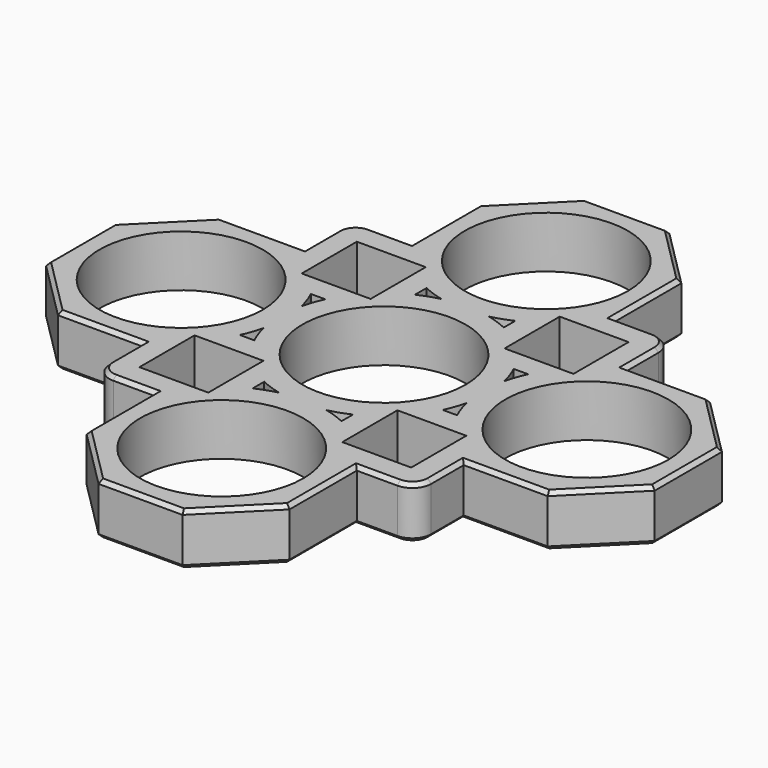
from build123d import *

# Parameters (mm, degrees)
F0_R         = 11.0109
F1_DEPTH     = 6.985
F2_W         = 9.299216499
F2_H         = 9.299216499
F3_DEPTH     = 25.4
F4_R         = 2.54
F5_SIZE      = 0.508
F6_SIZE      = 0.508
F7_T         = 3.048
F7_T3_DEPTH  = 12.065
F7_T5_DEPTH  = 6.9758818102
F7_T7_DEPTH  = 6.9758818102
F7_T9_DEPTH  = 6.9758818102
F7_T11_DEPTH = 6.9758818102
F7_T13_DEPTH = 6.9758818102
F7_T15_DEPTH = 13.081
F7_T17_DEPTH = 6.9758818102
F7_T19_DEPTH = 6.9758818102
F7_T21_DEPTH = 6.9758818102


# Not quite as in the source:
# - a shell that OpenCascade refuses in one call is made with other operations: the cavity is built on its own and cut out


with BuildPart() as f1:
    # F0 (on Top) → F1 (new body)
    with BuildSketch(Plane.XY):
        Polygon((-13.6927261634, 5.6717128827), (-13.6927261634, -5.6717128827), (-21.7137394441, -13.6927261634), (-21.7137394441, -21.7137394441), (-13.6927261634, -21.7137394441), (-5.6717128827, -13.6927261634), (5.6717128827, -13.6927261634), (13.6927261634, -21.7137394441), (21.7137394441, -21.7137394441), (21.7137394441, -13.6927261634), (13.6927261634, -5.6717128827), (13.6927261634, 5.6717128827), (21.7137394441, 13.6927261634), (21.7137394441, 21.7137394441), (13.6927261634, 21.7137394441), (5.6717128827, 13.6927261634), (-5.6717128827, 13.6927261634), (-13.6927261634, 21.7137394441), (-21.7137394441, 21.7137394441), (-21.7137394441, 13.6927261634), align=None)
        Circle(F0_R, mode=Mode.SUBTRACT)
        Polygon((-21.7137394441, -13.6927261634), (-13.6927261634, -5.6717128827), (-13.6927261634, 5.6717128827), (-21.7137394441, 13.6927261634), (-33.0571652095, 13.6927261634), (-41.0781784902, 5.6717128827), (-41.0781784902, -5.6717128827), (-33.0571652095, -13.6927261634), align=None)
        with Locations((-27.3854523268, 0)):
            Circle(F0_R, mode=Mode.SUBTRACT)
        Polygon((-5.6717128827, -13.6927261634), (-13.6927261634, -21.7137394441), (-13.6927261634, -33.0571652095), (-5.6717128827, -41.0781784902), (5.6717128827, -41.0781784902), (13.6927261634, -33.0571652095), (13.6927261634, -21.7137394441), (5.6717128827, -13.6927261634), align=None)
        with Locations((0, -27.3854523268)):
            Circle(F0_R, mode=Mode.SUBTRACT)
        Polygon((-13.6927261634, 33.0571652095), (-13.6927261634, 21.7137394441), (-5.6717128827, 13.6927261634), (5.6717128827, 13.6927261634), (13.6927261634, 21.7137394441), (13.6927261634, 33.0571652095), (5.6717128827, 41.0781784902), (-5.6717128827, 41.0781784902), align=None)
        with Locations((0, 27.3854523268)):
            Circle(F0_R, mode=Mode.SUBTRACT)
        Polygon((13.6927261634, -5.6717128827), (21.7137394441, -13.6927261634), (33.0571652095, -13.6927261634), (41.0781784902, -5.6717128827), (41.0781784902, 5.6717128827), (33.0571652095, 13.6927261634), (21.7137394441, 13.6927261634), (13.6927261634, 5.6717128827), align=None)
        with Locations((27.3854523268, 0)):
            Circle(F0_R, mode=Mode.SUBTRACT)
    extrude(amount=-F1_DEPTH)

    # F2 (on Top) → F3 (cut)
    with BuildSketch(Plane.XY):
        with Locations((-13.6927261634, 13.6927261634)):
            Rectangle(F2_W, F2_H)
        with Locations((13.6927261634, 13.6927261634)):
            Rectangle(F2_W, F2_H)
        with Locations((13.6927261634, -13.6927261634)):
            Rectangle(F2_W, F2_H)
        with Locations((-13.6927261634, -13.6927261634)):
            Rectangle(F2_W, F2_H)
    extrude(amount=-F3_DEPTH, mode=Mode.SUBTRACT)

    # F4
    f4_edges = [f1.edges().sort_by_distance(p)[0] for p in [
        (-21.713739, 21.713739, -3.4925),
        (21.713739, 21.713739, -3.4925),
        (21.713739, -21.713739, -3.4925),
        (-21.713739, -21.713739, -3.4925),
    ]]
    fillet(f4_edges, radius=F4_R)

    # F5
    f5_edges = [f1.edges().sort_by_distance(p)[0] for p in [
        (41.078178, 0, -6.985),
        (37.067672, 9.68222, -6.985),
        (27.385452, 13.692726, -6.985),
        (21.713739, 16.433233, -6.985),
        (16.433233, 21.713739, -6.985),
        (13.692726, 27.385452, -6.985),
        (9.68222, 37.067672, -6.985),
        (0, 41.078178, -6.985),
        (-9.68222, 37.067672, -6.985),
        (-13.692726, 27.385452, -6.985),
        (-16.433233, 21.713739, -6.985),
        (37.067672, -9.68222, -6.985),
        (27.385452, -13.692726, -6.985),
        (21.713739, -16.433233, -6.985),
        (16.433233, -21.713739, -6.985),
        (13.692726, -27.385452, -6.985),
        (9.68222, -37.067672, -6.985),
        (0, -41.078178, -6.985),
        (-9.68222, -37.067672, -6.985),
        (-13.692726, -27.385452, -6.985),
        (-16.433233, -21.713739, -6.985),
        (-21.713739, -16.433233, -6.985),
        (-27.385452, -13.692726, -6.985),
        (-37.067672, -9.68222, -6.985),
        (-41.078178, 0, -6.985),
        (-37.067672, 9.68222, -6.985),
        (-27.385452, 13.692726, -6.985),
        (-21.713739, 16.433233, -6.985),
    ]]
    chamfer(f5_edges, length=F5_SIZE)

    # F6
    f6_edges = [f1.edges().sort_by_distance(p)[0] for p in [
        (9.68222, -37.067672, 0),
        (0, -41.078178, 0),
        (-9.68222, -37.067672, 0),
        (-13.692726, -27.385452, 0),
        (-16.433233, -21.713739, 0),
        (-21.713739, -16.433233, 0),
        (-27.385452, -13.692726, 0),
        (-37.067672, -9.68222, 0),
        (-27.385452, 13.692726, 0),
        (-37.067672, 9.68222, 0),
        (-41.078178, 0, 0),
        (-21.713739, 16.433233, 0),
        (-16.433233, 21.713739, 0),
        (-13.692726, 27.385452, 0),
        (-9.68222, 37.067672, 0),
        (0, 41.078178, 0),
        (9.68222, 37.067672, 0),
        (13.692726, 27.385452, 0),
        (16.433233, 21.713739, 0),
        (21.713739, 16.433233, 0),
        (27.385452, 13.692726, 0),
        (37.067672, 9.68222, 0),
        (41.078178, 0, 0),
        (37.067672, -9.68222, 0),
        (27.385452, -13.692726, 0),
        (21.713739, -16.433233, 0),
        (16.433233, -21.713739, 0),
        (13.692726, -27.385452, 0),
    ]]
    chamfer(f6_edges, length=F6_SIZE)

    # F7: shell of thickness 3.048, made by hand


with BuildPart() as f7_core1:
    # F7_t2: copy of F1
    add(f1.part)

    # the walls: a layer under each face that stays
    f7_faces = [f7_core1.faces().sort_by_distance(p)[0] for p in [
        (21.7137394441, 16.4332328037, -3.4925),
        (21.4597394441, 16.1792328037, -0.254),
        (21.4597394441, 16.1792328037, -6.731),
        (27.3854523268, 13.6927261634, -3.4925),
        (20.7901855458, 20.7901855458, -0.254),
        (20.7901855458, 20.7901855458, -6.731),
        (16.4332328037, 21.7137394441, -3.4925),
        (27.1314523268, 13.4387261634, -0.254),
        (27.1314523268, 13.4387261634, -6.731),
        (37.0676718499, 9.6822195231, -3.4925),
        (16.1792328037, 21.4597394441, -0.254),
        (16.1792328037, 21.4597394441, -6.731),
        (13.6927261634, 27.3854523268, -3.4925),
        (36.8880667274, 9.5026144006, -0.254),
        (9.5026144006, -36.8880667274, -0.254),
        (0, -40.8241784902, -0.254),
        (13.4387261634, -27.1314523268, -0.254),
        (-9.5026144006, -36.8880667274, -0.254),
        (16.1792328037, -21.4597394441, -0.254),
        (-13.4387261634, -27.1314523268, -0.254),
        (20.7901855458, -20.7901855458, -0.254),
        (-16.1792328037, -21.4597394441, -0.254),
        (21.4597394441, -16.1792328037, -0.254),
        (-20.7901855458, -20.7901855458, -0.254),
        (27.1314523268, -13.4387261634, -0.254),
        (-21.4597394441, -16.1792328037, -0.254),
        (36.8880667274, -9.5026144006, -0.254),
        (-27.1314523268, -13.4387261634, -0.254),
        (40.8241784902, 0, -0.254),
        (-36.8880667274, -9.5026144006, -0.254),
        (-40.8241784902, 0, -0.254),
        (-36.8880667274, 9.5026144006, -0.254),
        (-27.1314523268, 13.4387261634, -0.254),
        (-21.4597394441, 16.1792328037, -0.254),
        (-20.7901855458, 20.7901855458, -0.254),
        (13.4387261634, 27.1314523268, -0.254),
        (-16.1792328037, 21.4597394441, -0.254),
        (9.5026144006, 36.8880667274, -0.254),
        (-13.4387261634, 27.1314523268, -0.254),
        (0, 40.8241784902, -0.254),
        (-9.5026144006, 36.8880667274, -0.254),
        (-9.0431179139, -13.6927261634, -3.4925),
        (-13.6927261634, -9.0431179139, -3.4925),
        (-18.3423344129, -13.6927261634, -3.4925),
        (-13.6927261634, -18.3423344129, -3.4925),
        (-11.0109, -27.3854523268, -3.4925),
        (18.3423344129, -13.6927261634, -3.4925),
        (13.6927261634, -9.0431179139, -3.4925),
        (9.0431179139, -13.6927261634, -3.4925),
        (13.6927261634, -18.3423344129, -3.4925),
        (-38.3963523268, 0, -3.4925),
        (-13.6927261634, 18.3423344129, -3.4925),
        (-18.3423344129, 13.6927261634, -3.4925),
        (-13.6927261634, 9.0431179139, -3.4925),
        (-9.0431179139, 13.6927261634, -3.4925),
        (-11.0109, 0, -3.4925),
        (9.0431179139, 13.6927261634, -3.4925),
        (13.6927261634, 9.0431179139, -3.4925),
        (18.3423344129, 13.6927261634, -3.4925),
        (13.6927261634, 18.3423344129, -3.4925),
        (16.3745523268, 0, -3.4925),
        (-11.0109, 27.3854523268, -3.4925),
        (36.8880667274, 9.5026144006, -6.731),
        (40.8241784902, 0, -6.731),
        (36.8880667274, -9.5026144006, -6.731),
        (27.1314523268, -13.4387261634, -6.731),
        (21.4597394441, -16.1792328037, -6.731),
        (20.7901855458, -20.7901855458, -6.731),
        (16.1792328037, -21.4597394441, -6.731),
        (13.4387261634, -27.1314523268, -6.731),
        (13.4387261634, 27.1314523268, -6.731),
        (9.5026144006, -36.8880667274, -6.731),
        (9.5026144006, 36.8880667274, -6.731),
        (0, -40.8241784902, -6.731),
        (0, 40.8241784902, -6.731),
        (-9.5026144006, -36.8880667274, -6.731),
        (-9.5026144006, 36.8880667274, -6.731),
        (-13.4387261634, -27.1314523268, -6.731),
        (-13.4387261634, 27.1314523268, -6.731),
        (-16.1792328037, -21.4597394441, -6.731),
        (-16.1792328037, 21.4597394441, -6.731),
        (-20.7901855458, -20.7901855458, -6.731),
        (-20.7901855458, 20.7901855458, -6.731),
        (-21.4597394441, -16.1792328037, -6.731),
        (-21.4597394441, 16.1792328037, -6.731),
        (-27.1314523268, -13.4387261634, -6.731),
        (-27.1314523268, 13.4387261634, -6.731),
        (-36.8880667274, -9.5026144006, -6.731),
        (-36.8880667274, 9.5026144006, -6.731),
        (-40.8241784902, 0, -6.731),
        (41.0781784902, 0, -3.4925),
        (9.6822195231, 37.0676718499, -3.4925),
        (9.6822195231, -37.0676718499, -3.4925),
        (0, -41.0781784902, -3.4925),
        (13.6927261634, -27.3854523268, -3.4925),
        (-9.6822195231, -37.0676718499, -3.4925),
        (16.4332328037, -21.7137394441, -3.4925),
        (-13.6927261634, -27.3854523268, -3.4925),
        (-16.4332328037, -21.7137394441, -3.4925),
        (21.7137394441, -16.4332328037, -3.4925),
        (27.3854523268, -13.6927261634, -3.4925),
        (-21.7137394441, -16.4332328037, -3.4925),
        (37.0676718499, -9.6822195231, -3.4925),
        (-27.3854523268, -13.6927261634, -3.4925),
        (-37.0676718499, -9.6822195231, -3.4925),
        (-41.0781784902, 0, -3.4925),
        (-37.0676718499, 9.6822195231, -3.4925),
        (-27.3854523268, 13.6927261634, -3.4925),
        (-21.7137394441, 16.4332328037, -3.4925),
        (-16.4332328037, 21.7137394441, -3.4925),
        (-13.6927261634, 27.3854523268, -3.4925),
        (0, 41.0781784902, -3.4925),
        (-9.6822195231, 37.0676718499, -3.4925),
    ]]
    thicken(f7_faces, amount=-F7_T, mode=Mode.SUBTRACT)

    # F7_s4 → F7_t3 (cut)
    with BuildSketch(Plane.XY.offset(-9.525)):
        Polygon((21.7442194441, 13.7232061634), (18.6657394441, 13.6927261634), (18.6657394441, 10.6447261634), (21.7137394441, 10.6447261634), align=None)
        Polygon((13.7232061634, 21.7442194441), (13.6927261634, 18.6657394441), (10.6447261634, 18.6657394441), (10.6447261634, 21.7137394441), align=None)
        Polygon((13.7232061634, -21.7442194441), (10.6447261634, -21.7137394441), (10.6447261634, -18.6657394441), (13.6927261634, -18.6657394441), align=None)
        Polygon((-13.7232061634, -21.7442194441), (-10.6447261634, -21.7137394441), (-10.6447261634, -18.6657394441), (-13.6927261634, -18.6657394441), align=None)
        Polygon((21.7442194441, -13.7232061634), (18.6657394441, -13.6927261634), (18.6657394441, -10.6447261634), (21.7137394441, -10.6447261634), align=None)
        Polygon((-21.7442194441, -13.7232061634), (-18.6657394441, -13.6927261634), (-18.6657394441, -10.6447261634), (-21.7137394441, -10.6447261634), align=None)
        Polygon((-21.7442194441, 13.7232061634), (-21.7137394441, 10.6447261634), (-18.6657394441, 10.6447261634), (-18.6657394441, 13.6927261634), align=None)
        Polygon((-13.7232061634, 21.7442194441), (-13.6927261634, 18.6657394441), (-10.6447261634, 18.6657394441), (-10.6447261634, 21.7137394441), align=None)
    extrude(amount=F7_T3_DEPTH, mode=Mode.SUBTRACT)

    # F7_s6 → F7_t5 (cut)
    with BuildSketch(Plane(origin=(9.7037249153, 9.7037249153, -9.7037249153), x_dir=(-0.7071067812, 0.7071067812, 0), z_dir=(0.5773502692, 0.5773502692, -0.5773502692))):
        Polygon((-5.6717128827, 14.0926417011), (-4.1477128827, 11.4002033618), (-5.6717128827, 10.5203215515), (-7.1957128827, 11.4002033618), align=None)
        Polygon((5.6717128827, 14.0926417011), (4.1477128827, 11.4002033618), (5.6717128827, 10.5203215515), (7.1957128827, 11.4002033618), align=None)
    extrude(amount=F7_T5_DEPTH, mode=Mode.SUBTRACT)

    # F7_s8 → F7_t7 (cut)
    with BuildSketch(Plane(origin=(11.402918823, 11.402918823, 11.402918823), x_dir=(0.7071067812, -0.7071067812, 0), z_dir=(-0.5773502692, -0.5773502692, -0.5773502692))):
        Polygon((5.6717128827, -19.7958703189), (4.1477128827, -17.1034319795), (5.6717128827, -16.2235501693), (7.1957128827, -17.1034319795), align=None)
        Polygon((-5.6717128827, -19.7958703189), (-4.1477128827, -17.1034319795), (-5.6717128827, -16.2235501693), (-7.1957128827, -17.1034319795), align=None)
    extrude(amount=F7_T7_DEPTH, mode=Mode.SUBTRACT)

    # F7_s10 → F7_t9 (cut)
    with BuildSketch(Plane(origin=(9.7037249153, -9.7037249153, -9.7037249153), x_dir=(0.7071067812, 0.7071067812, 0), z_dir=(0.5773502692, -0.5773502692, -0.5773502692))):
        Polygon((-5.6717128827, 14.0926417011), (-7.1957128827, 11.4002033618), (-5.6717128827, 10.5203215515), (-4.1477128827, 11.4002033618), align=None)
        Polygon((5.6717128827, 14.0926417011), (4.1477128827, 11.4002033618), (5.6717128827, 10.5203215515), (7.1957128827, 11.4002033618), align=None)
    extrude(amount=F7_T9_DEPTH, mode=Mode.SUBTRACT)

    # F7_s12 → F7_t11 (cut)
    with BuildSketch(Plane(origin=(-9.7037249153, -9.7037249153, -9.7037249153), x_dir=(0.7071067812, -0.7071067812, 0), z_dir=(-0.5773502692, -0.5773502692, -0.5773502692))):
        Polygon((5.6717128827, 14.0926417011), (7.1957128827, 11.4002033618), (5.6717128827, 10.5203215515), (4.1477128827, 11.4002033618), align=None)
        Polygon((-5.6717128827, 14.0926417011), (-4.1477128827, 11.4002033618), (-5.6717128827, 10.5203215515), (-7.1957128827, 11.4002033618), align=None)
    extrude(amount=F7_T11_DEPTH, mode=Mode.SUBTRACT)

    # F7_s14 → F7_t13 (cut)
    with BuildSketch(Plane(origin=(-9.7037249153, 9.7037249153, -9.7037249153), x_dir=(-0.7071067812, -0.7071067812, 0), z_dir=(-0.5773502692, 0.5773502692, -0.5773502692))):
        Polygon((5.6717128827, 14.0926417011), (7.1957128827, 11.4002033618), (5.6717128827, 10.5203215515), (4.1477128827, 11.4002033618), align=None)
        Polygon((-5.6717128827, 14.0926417011), (-4.1477128827, 11.4002033618), (-5.6717128827, 10.5203215515), (-7.1957128827, 11.4002033618), align=None)
    extrude(amount=F7_T13_DEPTH, mode=Mode.SUBTRACT)

    # F7_s16 → F7_t15 (cut)
    with BuildSketch(Plane.XY.offset(-10.033)):
        Polygon((-9.0735979139, -9.0735979139), (-5.9951179139, -9.0431179139), (-5.9951179139, -5.9951179139), (-9.0431179139, -5.9951179139), align=None)
        Polygon((-9.0735979139, -18.3118544129), (-5.9951179139, -18.3423344129), (-5.9951179139, -21.3903344129), (-9.0431179139, -21.3903344129), align=None)
        Polygon((-18.3118544129, -9.0735979139), (-18.3423344129, -5.9951179139), (-21.3903344129, -5.9951179139), (-21.3903344129, -9.0431179139), align=None)
        Polygon((-18.3118544129, -18.3118544129), (-21.3903344129, -18.3423344129), (-21.3903344129, -21.3903344129), (-18.3423344129, -21.3903344129), align=None)
        Polygon((18.3118544129, -9.0735979139), (21.3903344129, -9.0431179139), (21.3903344129, -5.9951179139), (18.3423344129, -5.9951179139), align=None)
        Polygon((18.3118544129, -18.3118544129), (21.3903344129, -18.3423344129), (21.3903344129, -21.3903344129), (18.3423344129, -21.3903344129), align=None)
        Polygon((9.0735979139, -9.0735979139), (9.0431179139, -5.9951179139), (5.9951179139, -5.9951179139), (5.9951179139, -9.0431179139), align=None)
        Polygon((9.0735979139, -18.3118544129), (5.9951179139, -18.3423344129), (5.9951179139, -21.3903344129), (9.0431179139, -21.3903344129), align=None)
        Polygon((-18.3118544129, 18.3118544129), (-18.3423344129, 21.3903344129), (-21.3903344129, 21.3903344129), (-21.3903344129, 18.3423344129), align=None)
        Polygon((-9.0735979139, 18.3118544129), (-9.0431179139, 21.3903344129), (-5.9951179139, 21.3903344129), (-5.9951179139, 18.3423344129), align=None)
        Polygon((-18.3118544129, 9.0735979139), (-21.3903344129, 9.0431179139), (-21.3903344129, 5.9951179139), (-18.3423344129, 5.9951179139), align=None)
        Polygon((-9.0735979139, 9.0735979139), (-9.0431179139, 5.9951179139), (-5.9951179139, 5.9951179139), (-5.9951179139, 9.0431179139), align=None)
        Polygon((9.0735979139, 9.0735979139), (5.9951179139, 9.0431179139), (5.9951179139, 5.9951179139), (9.0431179139, 5.9951179139), align=None)
        Polygon((9.0735979139, 18.3118544129), (5.9951179139, 18.3423344129), (5.9951179139, 21.3903344129), (9.0431179139, 21.3903344129), align=None)
        Polygon((18.3118544129, 9.0735979139), (18.3423344129, 5.9951179139), (21.3903344129, 5.9951179139), (21.3903344129, 9.0431179139), align=None)
        Polygon((18.3118544129, 18.3118544129), (21.3903344129, 18.3423344129), (21.3903344129, 21.3903344129), (18.3423344129, 21.3903344129), align=None)
    extrude(amount=F7_T15_DEPTH, mode=Mode.SUBTRACT)

    # F7_s18 → F7_t17 (cut)
    with BuildSketch(Plane(origin=(7.375391582, -7.375391582, 7.375391582), x_dir=(0.7071067812, 0.7071067812, 0), z_dir=(0.5773502692, -0.5773502692, 0.5773502692))):
        Polygon((5.6717128827, -19.7958703189), (7.1957128827, -17.1034319795), (5.6717128827, -16.2235501693), (4.1477128827, -17.1034319795), align=None)
        Polygon((-5.6717128827, -19.7958703189), (-4.1477128827, -17.1034319795), (-5.6717128827, -16.2235501693), (-7.1957128827, -17.1034319795), align=None)
    extrude(amount=F7_T17_DEPTH, mode=Mode.SUBTRACT)

    # F7_s20 → F7_t19 (cut)
    with BuildSketch(Plane(origin=(-7.375391582, -7.375391582, 7.375391582), x_dir=(0.7071067812, -0.7071067812, 0), z_dir=(-0.5773502692, -0.5773502692, 0.5773502692))):
        Polygon((5.6717128827, -19.7958703189), (7.1957128827, -17.1034319795), (5.6717128827, -16.2235501693), (4.1477128827, -17.1034319795), align=None)
        Polygon((-5.6717128827, -19.7958703189), (-4.1477128827, -17.1034319795), (-5.6717128827, -16.2235501693), (-7.1957128827, -17.1034319795), align=None)
    extrude(amount=F7_T19_DEPTH, mode=Mode.SUBTRACT)

    # F7_s22 → F7_t21 (cut)
    with BuildSketch(Plane(origin=(-7.375391582, 7.375391582, 7.375391582), x_dir=(-0.7071067812, -0.7071067812, 0), z_dir=(-0.5773502692, 0.5773502692, 0.5773502692))):
        Polygon((-5.6717128827, -19.7958703189), (-7.1957128827, -17.1034319795), (-5.6717128827, -16.2235501693), (-4.1477128827, -17.1034319795), align=None)
        Polygon((5.6717128827, -19.7958703189), (4.1477128827, -17.1034319795), (5.6717128827, -16.2235501693), (7.1957128827, -17.1034319795), align=None)
    extrude(amount=F7_T21_DEPTH, mode=Mode.SUBTRACT)


with BuildPart() as f1_1:
    add(f1.part)

    # what is left inside the walls is the cavity
    f7_cavity = [f7_core1.part.solids().sort_by_distance(p)[0] for p in [
        (13.307835, 4.627326, -4.656667),
        (4.627326, 14.077617, -4.656667),
        (-4.627326, 13.307835, -4.656667),
        (14.077617, -4.627326, -4.656667),
        (4.627326, -14.077617, -4.656667),
        (-4.627326, -13.307835, -4.656667),
        (-14.077617, 4.627326, -4.656667),
        (-14.077617, -4.627326, -4.656667),
    ]]
    add(f7_cavity, mode=Mode.SUBTRACT)


solid = f1_1.part
